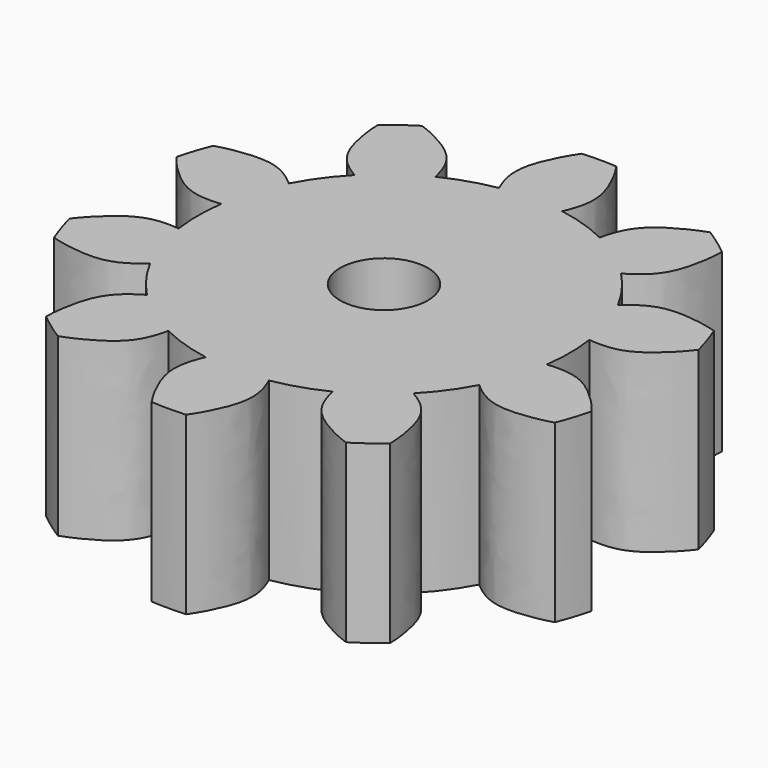
from build123d import *

# Parameters (mm, degrees)
F1_R     = 3
F2_DEPTH = 12
F3_COUNT = 10


# Not quite as in the source:
# - the dataset's text gives a spline's control points without its knots; the knots are read off the source's solid


with BuildPart() as f2:
    # F1 (on Top) → F2 (new body)
    with BuildSketch(Plane.XY):
        with BuildLine():
            add(Edge.make_bspline(
                [(1.1767889059, 18.3623301318), (1.6271784454, 17.7151013205), (2.818419618, 15.5665856482), (2.7289393763, 13.8155375104), (2.1532964325, 12.516122182)],
                knots=[0, 0, 0, 0, 0.4901902273, 1, 1, 1, 1], degree=3))
            ThreePointArc((1.1767889059, 18.3623301318), (0, 18.4), (-1.1767889059, 18.3623301318))
            add(Edge.make_bspline(
                [(-1.1767889059, 18.3623301318), (-1.6271784454, 17.7151013205), (-2.818419618, 15.5665856482), (-2.7289393763, 13.8155375104), (-2.1532964325, 12.516122182)],
                knots=[0, 0, 0, 0, 0.4901902273, 1, 1, 1, 1], degree=3))
            ThreePointArc((-2.1532964325, 12.516122182), (0, -12.7), (2.1532964325, 12.516122182))
        make_face()
        Circle(F1_R, mode=Mode.SUBTRACT)
    extrude(amount=F2_DEPTH)

    # F3: F2 ×10 about axis
    f3_axis = Axis((0, 0, 0), (0, 0, -1))


with BuildPart() as f2_1:
    add(f2.part)
    for i in range(1, F3_COUNT):
        add(f2.part.rotate(f3_axis, i * 360 / F3_COUNT))


solid = f2_1.part
